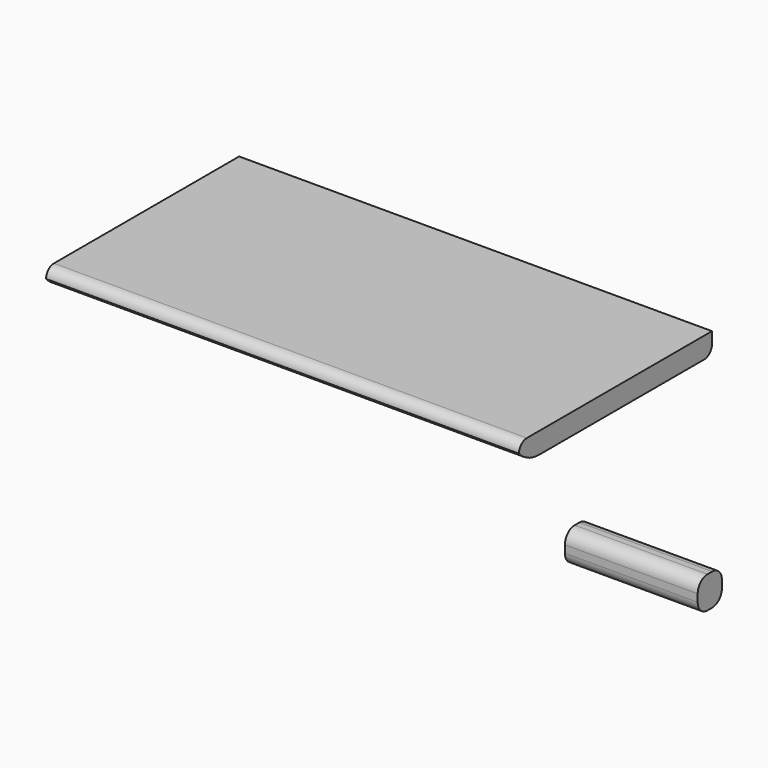
from build123d import *

# Parameters (mm, degrees)
F0_W        = 245.9494993091
F0_H        = 125.4998669028
F1_DEPTH    = 10.922
F2_R        = 5.08
F3_T1_DEPTH = 311.8374235671
F4_R        = 5.08
F5_W        = 69.0777301788
F5_H        = 16.571380198
F6_DEPTH    = 15.748
F7_R        = 6.35
F8_R        = 6.35
F9_R        = 6.35
F10_R       = 6.35


# Not quite as in the source:
# - a fillet or chamfer that OpenCascade refuses, or shapes differently, is made with other operations: its cross-section is extruded or revolved along the edge and cut away or added


with BuildPart() as f1:
    # F0 (on Top) → F1 (new body)
    with BuildSketch(Plane.XY):
        with Locations((9.6076615155, -14.3243558705)):
            Rectangle(F0_W, F0_H)
    extrude(amount=F1_DEPTH)

    # F2
    f2_edges = [f1.edges().sort_by_distance(p)[0] for p in [
        (9.607662, -77.074289, 10.922),
    ]]
    fillet(f2_edges, radius=F2_R)

    # F3: fillet of radius 17.7830971004 on 1 edges, made by hand

    # F3_s2 → F3_t1 (cut)
    with BuildSketch(Plane.YZ.offset(-146.3110502681)):
        with BuildLine():
            ThreePointArc((-77.0742893219, 5.842), (-71.1039526713, 1.5259720209), (-63.8967044703, 0))
            Line((-63.8967044703, 0), (-63.8967044703, -0.355661942))
            Line((-63.8967044703, -0.355661942), (-77.0742893219, -0.355661942))
            Line((-77.0742893219, -0.355661942), (-77.4299512639, 0))
            ThreePointArc((-77.4299512639, 0), (-77.4299512639, 2.921), (-77.3378410189, 5.603178058))
            Line((-77.3378410189, 5.603178058), (-77.0742893219, 5.842))
        make_face()
    extrude(amount=F3_T1_DEPTH, mode=Mode.SUBTRACT)

    # F4
    f4_edges = [f1.edges().sort_by_distance(p)[0] for p in [
        (9.607662, 48.425578, 0),
    ]]
    fillet(f4_edges, radius=F4_R)


with BuildPart() as f6:
    # F5 (on Front) → F6 (new body)
    with BuildSketch(Plane.XZ):
        with Locations((141.9334262609, -70.8999745548)):
            Rectangle(F5_W, F5_H)
    extrude(amount=F6_DEPTH)

    # F7
    f7_edges = [f6.edges().sort_by_distance(p)[0] for p in [
        (141.933426, 0, -79.185665),
    ]]
    fillet(f7_edges, radius=F7_R)

    # F8
    f8_edges = [f6.edges().sort_by_distance(p)[0] for p in [
        (141.933426, 0, -62.614284),
    ]]
    fillet(f8_edges, radius=F8_R)

    # F9
    f9_edges = [f6.edges().sort_by_distance(p)[0] for p in [
        (141.933426, -15.748, -79.185665),
    ]]
    fillet(f9_edges, radius=F9_R)

    # F10
    f10_edges = [f6.edges().sort_by_distance(p)[0] for p in [
        (141.933426, -15.748, -62.614284),
    ]]
    fillet(f10_edges, radius=F10_R)


solid = Compound([f1.part, f6.part])
